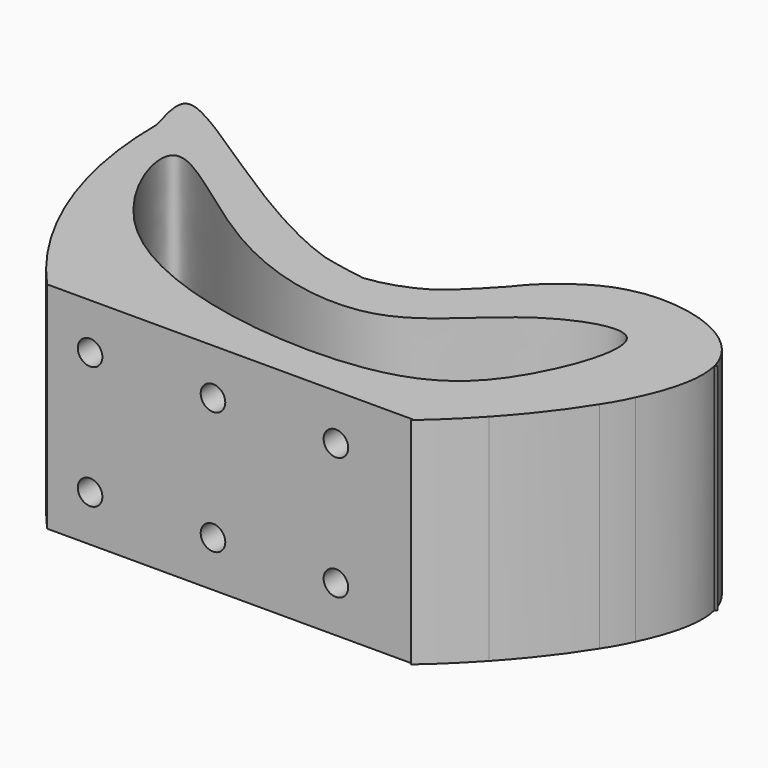
from build123d import *

# Parameters (mm, degrees)
F0_W      = 127
F0_H      = 127
F1_DEPTH  = 44.45
F3_W      = 5.52829355
F3_H      = 29.727132991
F3_W_2    = 15.5509337783
F3_H_2    = 31.797057949
F3_W_3    = 16.7360811029
F3_H_3    = 5.0730407238
F3_W_4    = 12.5154256821
F3_H_4    = 7.4998177588
F4_DEPTH  = 44.45
F6_DEPTH  = 44.45
F8_DEPTH  = 44.45
F10_DEPTH = 44.45
F11_DEPTH = 44.45
F13_DEPTH = 44.45
F14_W     = 40.5534765481
F14_H     = 44.45
F15_DEPTH = 25.4
F16_W     = 51.4885028824
F16_H     = 44.45
F17_DEPTH = 0.165514648
F18_W     = 20.4539634287
F18_H     = 44.45
F19_DEPTH = 0.5054324865
F20_W     = 63.3779155047
F20_H     = 44.45
F21_DEPTH = 0.1083666682
F22_DEPTH = 44.45
F24_DEPTH = 44.45
F25_W     = 75.4783482299
F25_H     = 21.748097633
F26_DEPTH = 44.45
F27_R     = 2.54
F28_DEPTH = 12.7
F30_DEPTH = 44.45


with BuildPart() as f1:
    # F0 (on Top) → F1 (new body)
    with BuildSketch(Plane.XY):
        Rectangle(F0_W, F0_H)
    extrude(amount=F1_DEPTH)

    # F3 (on face) → F4 (cut, through all)
    with BuildSketch(Plane.XY.offset(44.45)):
        Polygon((-42.7088961005, -20.6194780767), (-42.7088961005, 0), (-57.5702860951, 0), (-63.0985796452, 0), (-63.6439546943, 0), (-63.6439546943, -63.8658776879), (-42.7088961005, -63.8658776879), align=None)
        with Locations((-60.3344328701, 14.8635664955)):
            Rectangle(F3_W, F3_H)
        Polygon((47.7073714137, -20.6194780767), (-42.7088961005, -20.6194780767), (-42.7088961005, -63.8658776879), (63.258305192, -63.8658776879), (63.258305192, -24.8609110713), (63.258305192, -20.6194780767), align=None)
        with Locations((55.4828383029, -4.7209491022)):
            Rectangle(F3_W_2, F3_H_2)
        Polygon((15.835031867, 62.7080500126), (-35.6965474784, 62.7080500126), (-35.6965474784, 49.4633540511), (-20.397156477, 49.4633540511), (8.7539097294, 49.4633540511), (15.835031867, 49.4633540511), align=None)
        Polygon((8.7539097294, 49.4633540511), (-20.397156477, 49.4633540511), (-20.397156477, 42.0814976096), (-13.3289527148, 42.0814976096), (3.4071283881, 42.0814976096), (8.7539097294, 42.0814976096), align=None)
        with Locations((-4.9609121634, 39.5449772477)):
            Rectangle(F3_W_3, F3_H_3)
        with Locations((57.0145174861, 59.6473719925)):
            Rectangle(F3_W_4, F3_H_4)
    extrude(amount=-F4_DEPTH, mode=Mode.SUBTRACT)

    # F5 (on face) → F6 (cut, through all)
    with BuildSketch(Plane.XY.offset(44.45)):
        with BuildLine():
            ThreePointArc((-42.1748310328, 0), (-55.8025308374, 26.5772535751), (-63.3916333318, 55.4644502699))
            Line((-63.3916333318, 55.4644502699), (-63.3916333318, 0))
            Line((-63.3916333318, 0), (-42.1748310328, 0))
        make_face()
    extrude(amount=-F6_DEPTH, mode=Mode.SUBTRACT)

    # F7 (on face) → F8 (cut)
    with BuildSketch(Plane.XY.offset(44.45)):
        with BuildLine():
            ThreePointArc((-27.7672337737, -14.7277772986), (-34.772809099, -9.5105149668), (-40.4422940209, -2.8656031845))
            add(Edge.make_bspline(
                [(-40.4422940209, -2.8656031845), (-41.0425985075, -2.0697804555), (-41.6295465783, -1.2511429317), (-42.203463614, -0.4121370856)],
                knots=[0.7719634634, 0.7719634634, 0.7719634634, 0.7719634634, 0.7798458357, 0.7798458357, 0.7798458357, 0.7798458357], degree=3))
            Line((-42.203463614, -0.4121370856), (-42.203463614, -20.4539634287))
            Line((-42.203463614, -20.4539634287), (9.0681575239, -20.4539634287))
            Line((9.0681575239, -20.4539634287), (8.7691887717, -16.2410980862))
            add(Edge.make_bspline(
                [(8.7691887717, -16.2410980862), (8.5055559046, -16.3529711172), (8.2424805859, -16.4623264472), (7.9799670389, -16.5691767183)],
                knots=[0.6174011323, 0.6174011323, 0.6174011323, 0.6174011323, 0.6193995077, 0.6193995077, 0.6193995077, 0.6193995077], degree=3))
            ThreePointArc((7.9799670389, -16.5691767183), (1.6850007311, -18.7915432844), (-4.8966563137, -19.9083711648))
            add(Edge.make_bspline(
                [(-4.8966563137, -19.9083711648), (-13.3522734014, -20.7935789279), (-21.0357023958, -18.8874004708), (-27.7672337737, -14.7277772986)],
                knots=[0.6533615409, 0.6533615409, 0.6533615409, 0.6533615409, 0.7231284421, 0.7231284421, 0.7231284421, 0.7231284421], degree=3))
        make_face()
    extrude(amount=-F8_DEPTH, mode=Mode.SUBTRACT)

    # F9 (on face) → F10 (join, through all)
    with BuildSketch(Plane.XY.offset(44.45)):
        with BuildLine():
            ThreePointArc((53.1991496682, 22.8146277368), (33.6878318767, 0.2214438257), (8.7796067819, -16.2322428077))
            Line((8.7796067819, -16.2322428077), (8.7796067819, -20.729560405))
            Line((8.7796067819, -20.729560405), (67.3341974616, -23.1123883277))
            Line((67.3341974616, -23.1123883277), (67.3341974616, 48.1957755983))
            Line((67.3341974616, 48.1957755983), (59.4103001058, 44.9899025261))
            ThreePointArc((59.4103001058, 44.9899025261), (58.1087736986, 33.3969627769), (53.1991496682, 22.8146277368))
        make_face()
    extrude(amount=-F10_DEPTH)

    # F9 (on face) → F11 (cut)
    with BuildSketch(Plane.XY.offset(44.45)):
        with BuildLine():
            ThreePointArc((53.1991496682, 22.8146277368), (33.6878318767, 0.2214438257), (8.7796067819, -16.2322428077))
            Line((8.7796067819, -16.2322428077), (8.7796067819, -20.729560405))
            Line((8.7796067819, -20.729560405), (67.3341974616, -23.1123883277))
            Line((67.3341974616, -23.1123883277), (67.3341974616, 48.1957755983))
            Line((67.3341974616, 48.1957755983), (59.4103001058, 44.9899025261))
            ThreePointArc((59.4103001058, 44.9899025261), (58.1087736986, 33.3969627769), (53.1991496682, 22.8146277368))
        make_face()
    extrude(amount=-F11_DEPTH, mode=Mode.SUBTRACT)

    # F12 (on face) → F13 (cut)
    with BuildSketch(Plane.XY.offset(44.45)):
        with BuildLine():
            ThreePointArc((28.5480767488, 55.8399446309), (46.0439897256, 56.5803897157), (59.4402626157, 45.3023090959))
            Line((59.4402626157, 45.3023090959), (65.0680884719, 43.8909381628))
            Line((65.0680884719, 43.8909381628), (79.9444690347, 67.8006857634))
            Line((79.9444690347, 67.8006857634), (-66.2609507172, 66.0860144647))
            Line((-66.2609507172, 66.0860144647), (-63.1104335189, 62.9958063364))
            ThreePointArc((-63.1104335189, 62.9958063364), (-35.8684298989, 43.6042367441), (-3.9666965604, 33.582303673))
            ThreePointArc((-3.9666965604, 33.582303673), (6.5647988631, 37.0309720517), (14.9679081514, 44.255476445))
            ThreePointArc((14.9679081514, 44.255476445), (20.9580771779, 50.9854302577), (28.5480767488, 55.8399446309))
        make_face()
    extrude(amount=-F13_DEPTH, mode=Mode.SUBTRACT)

    # F14 (on face) → F15 (cut)
    with BuildSketch(Plane(origin=(63.258305192, 0, 0), x_dir=(0, -1, 0), z_dir=(-1, 0, 0))):
        with Locations((43.223261726, 22.225)):
            Rectangle(F14_W, F14_H)
    extrude(amount=-F15_DEPTH, mode=Mode.SUBTRACT)

    # F16 (on face) → F17 (cut, through all)
    with BuildSketch(Plane.XZ.offset(20.6194780767)):
        with Locations((-16.9646446593, 22.225)):
            Rectangle(F16_W, F16_H)
    extrude(amount=-F17_DEPTH, mode=Mode.SUBTRACT)

    # F18 (on face) → F19 (cut, through all)
    with BuildSketch(Plane(origin=(-42.7088961005, 0, 0), x_dir=(0, -1, 0), z_dir=(-1, 0, 0))):
        with Locations((10.2269817144, 22.225)):
            Rectangle(F18_W, F18_H)
    extrude(amount=-F19_DEPTH, mode=Mode.SUBTRACT)

    # F20 (on face) → F21 (cut, through all)
    with BuildSketch(Plane(origin=(-63.5, 0, 0), x_dir=(0, -1, 0), z_dir=(-1, 0, 0))):
        with Locations((-31.6889577524, 22.225)):
            Rectangle(F20_W, F20_H)
    extrude(amount=-F21_DEPTH, mode=Mode.SUBTRACT)

    # F2 (on face) → F22 (join)
    with BuildSketch(Plane.XY.offset(44.45)):
        with BuildLine():
            add(Edge.make_bspline(
                [(-63.5, 63.5), (-56.5301288519, 62.9660103461), (3.0846031043, 11.2650555358), (21.3203858799, 65.9622727195), (82.9524294609, 48.8490523279), (10.1216295014, -31.7931676724), (-29.0965706168, -18.3642097281), (-41.4307292783, -1.5622723401), (-42.4832404343, 0)],
                knots=[0, 0, 0, 0, 0.1732298849, 0.3066234834, 0.4281528556, 0.6173615434, 0.7665682512, 0.7811314402, 0.7811314402, 0.7811314402, 0.7811314402], degree=3))
            add(Edge.make_bspline(
                [(-63.5, 54.4128492475), (-65.004442094, 59.9811333867), (-66.0748426777, 63.6972689769), (-63.5, 63.5)],
                knots=[0.9360045988, 0.9360045988, 0.9360045988, 0.9360045988, 1, 1, 1, 1], degree=3))
            add(Edge.make_bspline(
                [(-42.4832404343, 0), (-53.6762372227, 16.6140845027), (-59.8591493369, 40.9372285625), (-63.5, 54.4128492475)],
                knots=[0.7811314402, 0.7811314402, 0.7811314402, 0.7811314402, 0.9360045988, 0.9360045988, 0.9360045988, 0.9360045988], degree=3))
        make_face()
        with BuildLine():
            Line((-63.5, 0), (-42.4832404343, 0))
            add(Edge.make_bspline(
                [(-42.4832404343, 0), (-53.6762372227, 16.6140845027), (-59.8591493369, 40.9372285625), (-63.5, 54.4128492475)],
                knots=[0.7811314402, 0.7811314402, 0.7811314402, 0.7811314402, 0.9360045988, 0.9360045988, 0.9360045988, 0.9360045988], degree=3))
            Line((-63.5, 54.4128492475), (-63.5, 0))
        make_face()
    extrude(amount=-F22_DEPTH)

    # F23 (on face) → F24 (cut)
    with BuildSketch(Plane.XY.offset(44.45)):
        with BuildLine():
            ThreePointArc((-42.4832404343, 0), (-58.0632295995, 25.2475344632), (-63.5, 54.4128492475))
            Line((-63.5, 54.4128492475), (-63.5, 0))
            Line((-63.5, 0), (-42.4832404343, 0))
        make_face()
    extrude(amount=-F24_DEPTH, mode=Mode.SUBTRACT)

    # F25 (on face) → F26 (cut)
    with BuildSketch(Plane.XY.offset(44.45)):
        with Locations((-4.7440663193, -10.8740488165)):
            Rectangle(F25_W, F25_H)
    extrude(amount=-F26_DEPTH, mode=Mode.SUBTRACT)

    # F27 (on face) → F28 (cut)
    with BuildSketch(Plane.XZ):
        with Locations((-33.5932404343, 34.925)):
            Circle(F27_R)
        with Locations((-33.5932404343, 9.525)):
            Circle(F27_R)
        with Locations((-8.1932404343, 34.925)):
            Circle(F27_R)
        with Locations((-8.1932404343, 9.525)):
            Circle(F27_R)
        with Locations((17.2067595657, 34.925)):
            Circle(F27_R)
        with Locations((17.2067595657, 9.525)):
            Circle(F27_R)
    extrude(amount=-F28_DEPTH, mode=Mode.SUBTRACT)

    # F29 (on face) → F30 (cut, through all)
    with BuildSketch(Plane.XY.offset(44.45)):
        with BuildLine():
            add(Edge.make_bspline(
                [(-54.6802394092, 47.9662790895), (-51.6145466363, 50.0460226855), (-27.5804482165, 27.42239441), (7.9438522494, 19.7535780522), (23.1109683336, 40.9498229071), (48.0346161993, 49.6086612554), (38.1114256694, 19.5679278095), (17.7429351354, 4.1864856123), (-45.9313308916, 12.5215588165), (-57.5578304123, 46.0141423608), (-54.6802394092, 47.9662790895)],
                knots=[0, 0, 0, 0, 0.128656713, 0.2661094932, 0.3817406077, 0.4753631519, 0.5814878035, 0.6986401594, 0.8792372794, 1, 1, 1, 1], degree=3))
        make_face()
    extrude(amount=-F30_DEPTH, mode=Mode.SUBTRACT)


solid = f1.part
